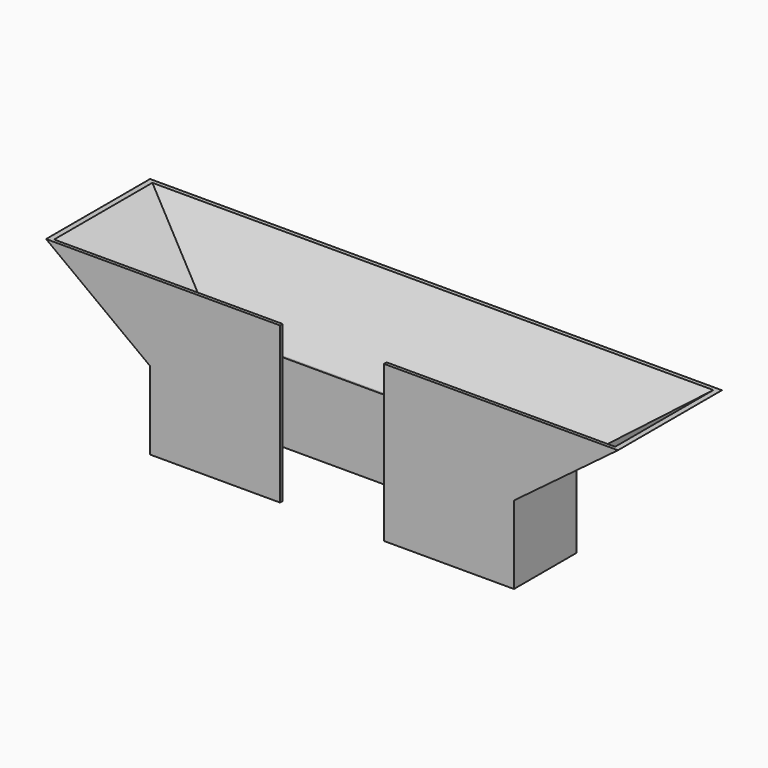
from build123d import *

# Parameters (mm, degrees)
F1_DEPTH    = 355.6
F2_W        = 355.6
F2_H        = 76.2
F3_DEPTH    = 127
F5_DEPTH    = 457.201
F6_DEPTH    = 101.601
F7_T        = 3.175
F7_T3_DEPTH = 82.55
F7_T5_DEPTH = 361.95
F8_W        = 101.6
F8_H        = 228.6
F9_DEPTH    = 25.4


# Not quite as in the source:
# - a shell that OpenCascade refuses in one call is made with other operations: the cavity is built on its own and cut out


with BuildPart() as f1:
    # F0 (on Right) → F1 (new body)
    with BuildSketch(Plane.YZ):
        Polygon((0, 152.4), (0, 0), (76.2, 0), (76.2, 76.2), (76.2, 152.4), align=None)
        Polygon((76.2, 152.4), (76.2, 76.2), (127, 152.4), align=None)
    extrude(amount=F1_DEPTH)

    # F2 (on face) → F3 (join)
    with BuildSketch(Plane.XZ):
        Polygon((457.2, 152.4), (355.6, 152.4), (355.6, 76.2), align=None)
        Polygon((0, 76.2), (0, 152.4), (-101.6, 152.4), align=None)
        with Locations((177.8, 114.3)):
            Rectangle(F2_W, F2_H)
    extrude(amount=-F3_DEPTH)

    # F4 (on face) → F5 (cut, through all)
    with BuildSketch(Plane.YZ.offset(355.6)):
        Polygon((76.2, 76.2), (127, 76.2), (127, 152.4), align=None)
    extrude(amount=-F5_DEPTH, mode=Mode.SUBTRACT)

    # F4 (on face) → F6 (cut, through all)
    with BuildSketch(Plane.YZ.offset(355.6)):
        Polygon((76.2, 76.2), (127, 76.2), (127, 152.4), align=None)
    extrude(amount=F6_DEPTH, mode=Mode.SUBTRACT)

    # F7: shell of thickness 3.175, made by hand


with BuildPart() as f7_core1:
    # F7_t2: copy of F1
    add(f1.part)

    # the walls: a layer under each face that stays
    f7_faces = [f7_core1.faces().sort_by_distance(p)[0] for p in [
        (177.8, 0, 76.2),
        (-50.8, 63.5, 114.3),
        (177.8, 101.6, 114.3),
        (177.8, 76.2, 38.1),
        (0, 38.1, 38.1),
        (355.6, 38.1, 38.1),
        (406.4, 63.5, 114.3),
    ]]
    thicken(f7_faces, amount=-F7_T, mode=Mode.SUBTRACT)

    # F7_s4 → F7_t3 (cut)
    with BuildSketch(Plane.XZ.offset(-79.375)):
        Polygon((-0.0508, 76.1746), (1.905, 78.74), (3.175, 77.7875), (3.175, 76.2), align=None)
        Polygon((355.6508, 76.1746), (352.425, 76.2), (352.425, 77.7875), (353.695, 78.74), align=None)
    extrude(amount=F7_T3_DEPTH, mode=Mode.SUBTRACT)

    # F7_s6 → F7_t5 (cut)
    with BuildSketch(Plane.YZ.offset(-3.175)):
        Polygon((76.2581675968, 76.1823882688), (73.5582403155, 77.961173123), (73.025, 77.1613126498), (73.025, 76.2), align=None)
    extrude(amount=F7_T5_DEPTH, mode=Mode.SUBTRACT)


with BuildPart() as f1_1:
    add(f1.part)

    # what is left inside the walls is the cavity
    f7_cavity = [f7_core1.part.solids().sort_by_distance(p)[0] for p in [
        (269.169444, 63.179562, 152.36825),
    ]]
    add(f7_cavity, mode=Mode.SUBTRACT)

    # F8 (on face) → F9 (cut)
    with BuildSketch(Plane.XZ):
        with Locations((177.8, 38.1)):
            Rectangle(F8_W, F8_H)
    extrude(amount=-F9_DEPTH, mode=Mode.SUBTRACT)


solid = f1_1.part
